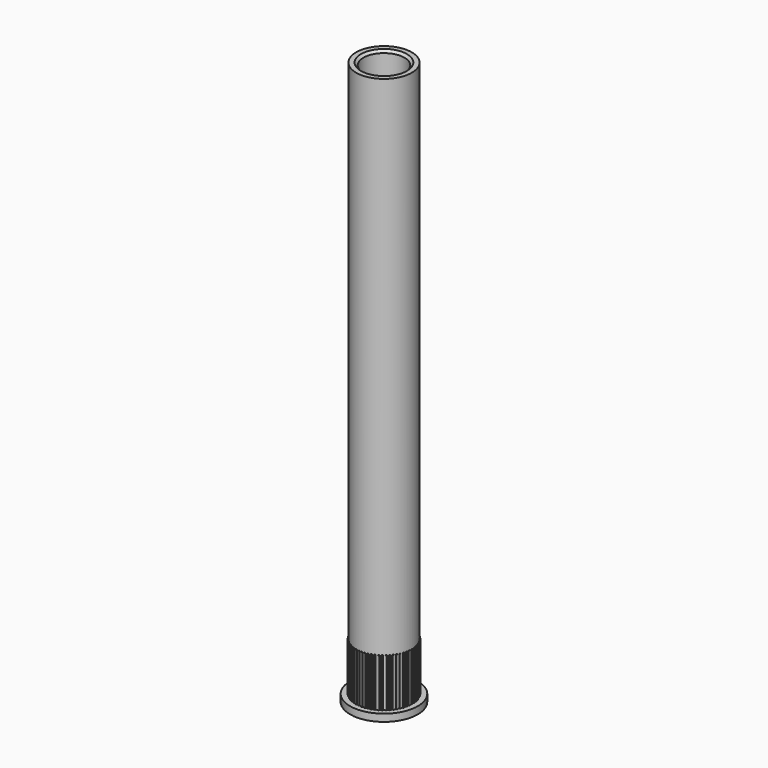
from build123d import *

# Parameters (mm, degrees)
F2_R            = 0.25
F3_DEPTH        = 20
F3_COPIES_COUNT = 60
F4_SIZE         = 1


# Not quite as in the source:
# - a pattern or mirror of a feature is missing from the dataset's text; its kind, count and spacing are read off the source's solid


with BuildPart() as f1:
    # F0 (on Front) → F1 (revolve)
    with BuildSketch(Plane.XZ):
        Polygon((-14, 0), (-8.5, 0), (-8.5, 233), (-11.5, 233), (-11.5, 3), (-14, 3), align=None)
    revolve(axis=Axis((0, 0, 48.0585359184), (0, 0, 1)))

    # F2 (on face) → F3 (join)
    with BuildSketch(Plane.XY.offset(3)):
        with Locations((0, -11.5)):
            Circle(F2_R)
    f3 = extrude(amount=F3_DEPTH)

    # F3_copies: F3 ×60 about axis
    f3_copies_axis = Axis((0, 0, 0), (0, 0, 1))
    for i in range(1, F3_COPIES_COUNT):
        add(f3.rotate(f3_copies_axis, i * 360 / F3_COPIES_COUNT))

    # F4
    f4_edges = [f1.edges().sort_by_distance(p)[0] for p in [
        (8.5, 0, 0),
        (8.5, 0, 233),
    ]]
    chamfer(f4_edges, length=F4_SIZE)


solid = f1.part
